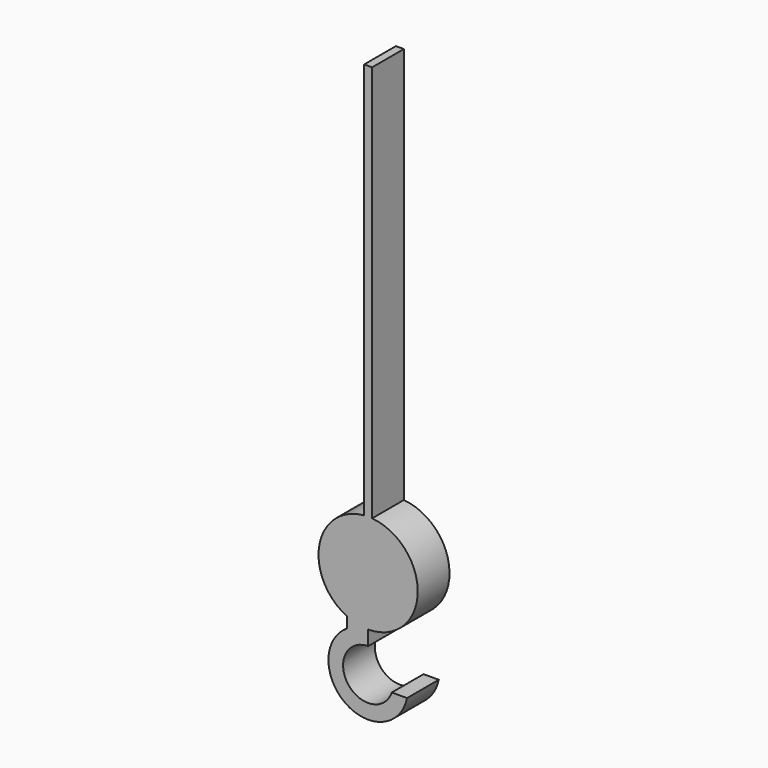
from build123d import *

# Parameters (mm, degrees)
F1_DEPTH = 60.96


# Not quite as in the source:
# - a feature names something its author has since deleted; it is built from what else it names


with BuildPart() as f1:
    # F0 (on Front) → F1 (new body)
    with BuildSketch(Plane.XZ):
        with BuildLine():
            Line((-6.096, 685.5557686025), (-6.096, 75.9557686025))
            ThreePointArc((-6.096, 75.9557686025), (-74.9833545956, 13.5623203614), (-32.3157872997, -69.0081871317))
            Line((-32.3157872997, -69.0081871317), (-32.3157872997, -85.470431505))
            ThreePointArc((-32.3157872997, -85.470431505), (-34.8273647694, -187.19175255), (59.6940359728, -149.5189509783))
            Line((59.6940359728, -149.5189509783), (36.3618585551, -149.5189509783))
            ThreePointArc((36.3618585551, -149.5189509783), (-31.2215584924, -159.5238706884), (0, -98.7552030748))
            Line((0, -98.7552030748), (0, -76.2))
            ThreePointArc((0, -76.2), (76.1389176687, -3.0504452534), (6.096, 75.9557686025))
            Line((6.096, 75.9557686025), (6.096, 685.5557686025))
            Line((6.096, 685.5557686025), (-6.096, 685.5557686025))
        make_face()
    extrude(amount=F1_DEPTH)


solid = f1.part
